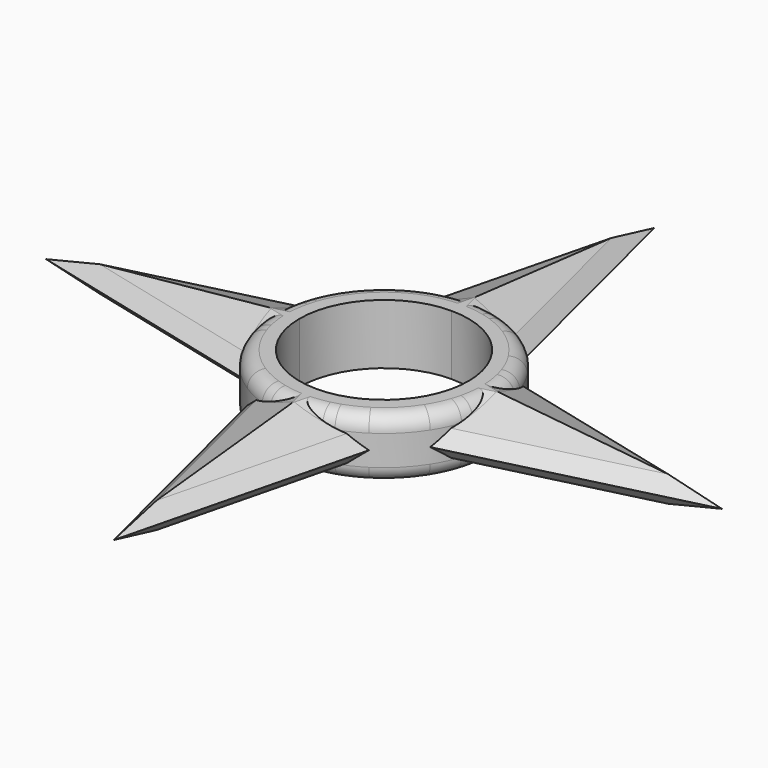
from build123d import *

# Parameters (mm, degrees)
F1_DEPTH      = 203.2
F2_SIZE       = 101.59999
F3_SIZE       = 81.28
F4_T2_ANGLE   = 24.7002002524
F4_T4_ANGLE   = 24.7002002524
F4_T6_ANGLE   = 24.7002002524
F4_T8_ANGLE   = 24.7002002524
F4_T10_ANGLE  = 24.7002002524
F4_T12_ANGLE  = 24.7002002524
F4_T14_ANGLE  = 24.7002002524
F4_T16_ANGLE  = 24.7002002524
F4_T20_ANGLE  = 19.2383475562
F4_T25_ANGLE  = 19.2383475562
F4_T30_ANGLE  = 19.2383475562
F4_T35_ANGLE  = 19.2383475562
F4_T40_ANGLE  = 19.2383475562
F4_T45_ANGLE  = 19.2383475562
F4_T50_ANGLE  = 19.2383475562
F4_T55_ANGLE  = 19.2383475562
F4_T60_ANGLE  = 19.2383475562
F4_T65_ANGLE  = 19.2383475562
F4_T70_ANGLE  = 19.2383475562
F4_T75_ANGLE  = 19.2383475562
F4_T80_ANGLE  = 19.2383475562
F4_T85_ANGLE  = 19.2383475562
F4_T90_ANGLE  = 19.2383475562
F4_T95_ANGLE  = 19.2383475562
F4_T100_ANGLE = 32.2106057484
F4_T105_ANGLE = 32.2106057484
F4_T110_ANGLE = 32.2106057484
F4_T115_ANGLE = 32.2106057484
F4_T120_ANGLE = 32.2106057484
F4_T125_ANGLE = 32.2106057484
F4_T130_ANGLE = 32.2106057484
F4_T135_ANGLE = 32.2106057484
F4_T140_ANGLE = 32.2106057484
F4_T145_ANGLE = 32.2106057484
F4_T150_ANGLE = 32.2106057484
F4_T155_ANGLE = 32.2106057484
F4_T160_ANGLE = 32.2106057484
F4_T165_ANGLE = 32.2106057484
F4_T170_ANGLE = 32.2106057484
F4_T175_ANGLE = 32.2106057484
F4_T180_ANGLE = 32.2106057484
F4_T185_ANGLE = 32.2106057484
F4_T190_ANGLE = 32.2106057484
F4_T195_ANGLE = 32.2106057484
F4_T200_ANGLE = 32.2106057484
F4_T205_ANGLE = 32.2106057484
F4_T210_ANGLE = 32.2106057484
F4_T215_ANGLE = 32.2106057484
F4_T220_ANGLE = 32.2106057484
F4_T225_ANGLE = 32.2106057484
F4_T230_ANGLE = 32.2106057484
F4_T235_ANGLE = 32.2106057484
F4_T240_ANGLE = 32.2106057484
F4_T245_ANGLE = 32.2106057484
F4_T250_ANGLE = 32.2106057484
F4_T255_ANGLE = 32.2106057484


# Not quite as in the source:
# - a fillet or chamfer that OpenCascade refuses, or shapes differently, is made with other operations: its cross-section is extruded or revolved along the edge and cut away or added
# - a fillet or chamfer is up to 0.001 mm smaller than in the source, because OpenCascade refuses the exact size


with BuildPart() as f1:
    # F0 (on Top) → F1 (new body)
    with BuildSketch(Plane.XY):
        with BuildLine():
            ThreePointArc((-205.551133263, 320.7954669478), (-107.0932469693, 365.6392162413), (0, 381))
            Line((0, 381), (0, 1143))
            Line((0, 1143), (-190.5, 381))
            Line((-190.5, 381), (-205.551133263, 320.7954669478))
        make_face()
        with BuildLine():
            Line((0, 1143), (0, 381))
            ThreePointArc((0, 381), (107.0932469693, 365.6392162413), (205.551133263, 320.7954669478))
            Line((205.551133263, 320.7954669478), (190.5, 381))
            Line((190.5, 381), (0, 1143))
        make_face()
        with BuildLine():
            Line((-1143, 0), (-381, 0))
            ThreePointArc((-381, 0), (-365.6392162413, 107.0932469693), (-320.7954669478, 205.551133263))
            Line((-320.7954669478, 205.551133263), (-381, 190.5))
            Line((-381, 190.5), (-1143, 0))
        make_face()
        with BuildLine():
            ThreePointArc((-320.7954669478, -205.551133263), (-365.6392162413, -107.0932469693), (-381, 0))
            Line((-381, 0), (-1143, 0))
            Line((-1143, 0), (-381, -190.5))
            Line((-381, -190.5), (-320.7954669478, -205.551133263))
        make_face()
        with BuildLine():
            Line((0, -1143), (0, -381))
            ThreePointArc((0, -381), (-107.0932469693, -365.6392162413), (-205.551133263, -320.7954669478))
            Line((-205.551133263, -320.7954669478), (-190.5, -381))
            Line((-190.5, -381), (0, -1143))
        make_face()
        with BuildLine():
            ThreePointArc((205.551133263, -320.7954669478), (107.0932469693, -365.6392162413), (0, -381))
            Line((0, -381), (0, -1143))
            Line((0, -1143), (190.5, -381))
            Line((190.5, -381), (205.551133263, -320.7954669478))
        make_face()
        with BuildLine():
            Line((1143, 0), (381, 0))
            ThreePointArc((381, 0), (365.6392162413, -107.0932469693), (320.7954669478, -205.551133263))
            Line((320.7954669478, -205.551133263), (381, -190.5))
            Line((381, -190.5), (1143, 0))
        make_face()
        with BuildLine():
            ThreePointArc((320.7954669478, 205.551133263), (365.6392162413, 107.0932469693), (381, 0))
            Line((381, 0), (1143, 0))
            Line((1143, 0), (381, 190.5))
            Line((381, 190.5), (320.7954669478, 205.551133263))
        make_face()
        with BuildLine():
            ThreePointArc((0, 292.1), (206.5458907846, 206.5458907846), (292.1, 0))
            Line((292.1, 0), (381, 0))
            ThreePointArc((381, 0), (365.6392162413, 107.0932469693), (320.7954669478, 205.551133263))
            ThreePointArc((320.7954669478, 205.551133263), (269.4076836321, 269.4076836321), (205.551133263, 320.7954669478))
            ThreePointArc((205.551133263, 320.7954669478), (107.0932469693, 365.6392162413), (0, 381))
            Line((0, 381), (0, 292.1))
        make_face()
        with BuildLine():
            ThreePointArc((-292.1, 0), (-206.5458907846, 206.5458907846), (0, 292.1))
            Line((0, 292.1), (0, 381))
            ThreePointArc((0, 381), (-107.0932469693, 365.6392162413), (-205.551133263, 320.7954669478))
            ThreePointArc((-205.551133263, 320.7954669478), (-269.4076836321, 269.4076836321), (-320.7954669478, 205.551133263))
            ThreePointArc((-320.7954669478, 205.551133263), (-365.6392162413, 107.0932469693), (-381, 0))
            Line((-381, 0), (-292.1, 0))
        make_face()
        with BuildLine():
            Line((381, 0), (292.1, 0))
            ThreePointArc((292.1, 0), (206.5458907846, -206.5458907846), (0, -292.1))
            Line((0, -292.1), (0, -381))
            ThreePointArc((0, -381), (107.0932469693, -365.6392162413), (205.551133263, -320.7954669478))
            ThreePointArc((205.551133263, -320.7954669478), (269.4076836321, -269.4076836321), (320.7954669478, -205.551133263))
            ThreePointArc((320.7954669478, -205.551133263), (365.6392162413, -107.0932469693), (381, 0))
        make_face()
        with BuildLine():
            ThreePointArc((-292.1, 0), (-206.5458907846, -206.5458907846), (0, -292.1))
            Line((0, -292.1), (0, -285.75))
            ThreePointArc((0, -285.75), (-202.0557627241, -202.0557627241), (-285.75, 0))
            Line((-285.75, 0), (-292.1, 0))
        make_face()
        with BuildLine():
            Line((0, 285.75), (0, 292.1))
            ThreePointArc((0, 292.1), (-206.5458907846, 206.5458907846), (-292.1, 0))
            Line((-292.1, 0), (-285.75, 0))
            ThreePointArc((-285.75, 0), (-202.0557627241, 202.0557627241), (0, 285.75))
        make_face()
        with BuildLine():
            ThreePointArc((0, -292.1), (206.5458907846, -206.5458907846), (292.1, 0))
            Line((292.1, 0), (285.75, 0))
            ThreePointArc((285.75, 0), (202.0557627241, -202.0557627241), (0, -285.75))
            Line((0, -285.75), (0, -292.1))
        make_face()
        with BuildLine():
            Line((285.75, 0), (292.1, 0))
            ThreePointArc((292.1, 0), (206.5458907846, 206.5458907846), (0, 292.1))
            Line((0, 292.1), (0, 285.75))
            ThreePointArc((0, 285.75), (202.0557627241, 202.0557627241), (285.75, 0))
        make_face()
        with BuildLine():
            Line((0, -381), (0, -292.1))
            ThreePointArc((0, -292.1), (-206.5458907846, -206.5458907846), (-292.1, 0))
            Line((-292.1, 0), (-381, 0))
            ThreePointArc((-381, 0), (-365.6392162413, -107.0932469693), (-320.7954669478, -205.551133263))
            ThreePointArc((-320.7954669478, -205.551133263), (-269.4076836321, -269.4076836321), (-205.551133263, -320.7954669478))
            ThreePointArc((-205.551133263, -320.7954669478), (-107.0932469693, -365.6392162413), (0, -381))
        make_face()
    extrude(amount=F1_DEPTH)

    # F2 (size 101.6 in the source; OpenCascade refuses exactly that, so slightly less here)
    f2_edges = [f1.edges().sort_by_distance(p)[0] for p in [
        (-731.897733, -102.775567, 203.2),
        (-731.897733, -102.775567, 0),
        (-731.897733, 102.775567, 203.2),
        (-731.897733, 102.775567, 0),
        (-102.775567, 731.897733, 203.2),
        (-102.775567, 731.897733, 0),
        (102.775567, 731.897733, 203.2),
        (102.775567, 731.897733, 0),
        (731.897733, 102.775567, 203.2),
        (731.897733, 102.775567, 0),
        (731.897733, -102.775567, 203.2),
        (731.897733, -102.775567, 0),
        (102.775567, -731.897733, 203.2),
        (102.775567, -731.897733, 0),
        (-102.775567, -731.897733, 203.2),
        (-102.775567, -731.897733, 0),
    ]]
    chamfer(f2_edges, length=F2_SIZE)

    # F3
    f3_edges = [f1.edges().sort_by_distance(p)[0] for p in [
        (-44.185339, -547.351154, 203.2),
        (44.185339, -547.351154, 203.2),
        (547.351154, -44.185339, 203.2),
        (547.351154, 44.185339, 203.2),
        (44.185339, 547.351154, 203.2),
        (-44.185339, 547.351154, 203.2),
        (-547.351154, 44.185339, 203.2),
        (-547.351154, -44.185339, 203.2),
        (-44.185339, 547.351154, 0),
        (44.185339, 547.351154, 0),
        (547.351154, 44.185339, 0),
        (547.351154, -44.185339, 0),
        (44.185339, -547.351154, 0),
        (-44.185339, -547.351154, 0),
        (-547.351154, 44.185339, 0),
        (-547.351154, -44.185339, 0),
    ]]
    chamfer(f3_edges, length=F3_SIZE)

    # F4: fillet of radius 50.8 on 24 edges, made by hand

    # F4_s1 → F4_t2 (revolve, cut)
    with BuildSketch(Plane(origin=(0, 0, 0), x_dir=(0, 0, 1), z_dir=(0.8419828529, 0.5395042868, 0))):
        with BuildLine():
            ThreePointArc((0, -330.2), (14.8789755157, -366.1210244843), (50.8, -381))
            Line((50.8, -381), (0, -381))
            Line((0, -381), (0, -330.2))
        make_face()
    revolve(axis=Axis((0, 0, 0), (0, 0, 1)), revolution_arc=F4_T2_ANGLE, mode=Mode.SUBTRACT)

    # F4_s3 → F4_t4 (revolve, cut)
    with BuildSketch(Plane(origin=(0, 0, 0), x_dir=(0, 0, 1), z_dir=(0.8419828529, 0.5395042868, 0))):
        with BuildLine():
            ThreePointArc((203.2, -330.2), (188.3210244843, -366.1210244843), (152.4, -381))
            Line((152.4, -381), (203.2, -381))
            Line((203.2, -381), (203.2, -330.2))
        make_face()
    revolve(axis=Axis((0, 0, 203.2), (0, 0, 1)), revolution_arc=F4_T4_ANGLE, mode=Mode.SUBTRACT)

    # F4_s5 → F4_t6 (revolve, cut)
    with BuildSketch(Plane(origin=(0, 0, 0), x_dir=(0, 0, 1), z_dir=(0.5395042868, -0.8419828529, 0))):
        with BuildLine():
            ThreePointArc((0, -330.2), (14.8789755157, -366.1210244843), (50.8, -381))
            Line((50.8, -381), (0, -381))
            Line((0, -381), (0, -330.2))
        make_face()
    revolve(axis=Axis((0, 0, 0), (0, 0, 1)), revolution_arc=F4_T6_ANGLE, mode=Mode.SUBTRACT)

    # F4_s7 → F4_t8 (revolve, cut)
    with BuildSketch(Plane(origin=(0, 0, 0), x_dir=(0, 0, 1), z_dir=(0.5395042868, -0.8419828529, 0))):
        with BuildLine():
            ThreePointArc((203.2, -330.2), (188.3210244843, -366.1210244843), (152.4, -381))
            Line((152.4, -381), (203.2, -381))
            Line((203.2, -381), (203.2, -330.2))
        make_face()
    revolve(axis=Axis((0, 0, 203.2), (0, 0, 1)), revolution_arc=F4_T8_ANGLE, mode=Mode.SUBTRACT)

    # F4_s9 → F4_t10 (revolve, cut)
    with BuildSketch(Plane(origin=(0, 0, 0), x_dir=(0, 0, 1), z_dir=(-0.8419828529, -0.5395042868, 0))):
        with BuildLine():
            ThreePointArc((0, -330.2), (14.8789755157, -366.1210244843), (50.8, -381))
            Line((50.8, -381), (0, -381))
            Line((0, -381), (0, -330.2))
        make_face()
    revolve(axis=Axis((0, 0, 0), (0, 0, 1)), revolution_arc=F4_T10_ANGLE, mode=Mode.SUBTRACT)

    # F4_s11 → F4_t12 (revolve, cut)
    with BuildSketch(Plane(origin=(0, 0, 0), x_dir=(0, 0, 1), z_dir=(-0.8419828529, -0.5395042868, 0))):
        with BuildLine():
            ThreePointArc((203.2, -330.2), (188.3210244843, -366.1210244843), (152.4, -381))
            Line((152.4, -381), (203.2, -381))
            Line((203.2, -381), (203.2, -330.2))
        make_face()
    revolve(axis=Axis((0, 0, 203.2), (0, 0, 1)), revolution_arc=F4_T12_ANGLE, mode=Mode.SUBTRACT)

    # F4_s13 → F4_t14 (revolve, cut)
    with BuildSketch(Plane(origin=(0, 0, 0), x_dir=(0, 0, 1), z_dir=(-0.5395042868, 0.8419828529, 0))):
        with BuildLine():
            ThreePointArc((50.8, -381), (14.8789755157, -366.1210244843), (0, -330.2))
            Line((0, -330.2), (0, -381))
            Line((0, -381), (50.8, -381))
        make_face()
    revolve(axis=Axis((0, 0, 0), (0, 0, 1)), revolution_arc=F4_T14_ANGLE, mode=Mode.SUBTRACT)

    # F4_s15 → F4_t16 (revolve, cut)
    with BuildSketch(Plane(origin=(0, 0, 0), x_dir=(0, 0, 1), z_dir=(-0.5395042868, 0.8419828529, 0))):
        with BuildLine():
            ThreePointArc((152.4, -381), (188.3210244843, -366.1210244843), (203.2, -330.2))
            Line((203.2, -330.2), (203.2, -381))
            Line((203.2, -381), (152.4, -381))
        make_face()
    revolve(axis=Axis((0, 0, 203.2), (0, 0, 1)), revolution_arc=F4_T16_ANGLE, mode=Mode.SUBTRACT)


with BuildPart() as f4_tool18:
    # F4_s19 → F4_t20 (revolve)
    with BuildSketch(Plane(origin=(0, 0, 0), x_dir=(0, 0, 1), z_dir=(0.5395042868, -0.8419828529, 0))):
        with BuildLine():
            ThreePointArc((50.8, 381), (14.8789755157, 366.1210244843), (0, 330.2))
            Line((0, 330.2), (0, 381))
            Line((0, 381), (50.8, 381))
        make_face()
    revolve(axis=Axis((0, 0, 0), (0, 0, -1)), revolution_arc=F4_T20_ANGLE)

    split(bisect_by=Plane(origin=(-3.3507542833, -13.4030171331, -33.3536008728), x_dir=(0.9701425001, -0.242535625, 0), z_dir=(-0.0928143655, -0.3712574618, -0.9238795325)), keep=Keep.TOP)


with BuildPart() as f1_1:
    add(f1.part)

    # F4_t17: cut F4_tool18
    add(f4_tool18.part, mode=Mode.SUBTRACT)


with BuildPart() as f4_tool23:
    # F4_s24 → F4_t25 (revolve)
    with BuildSketch(Plane(origin=(0, 0, 0), x_dir=(0, 0, 1), z_dir=(-0.8419828529, 0.5395042868, 0))):
        with BuildLine():
            ThreePointArc((50.8, -381), (14.8789755157, -366.1210244843), (0, -330.2))
            Line((0, -330.2), (0, -381))
            Line((0, -381), (50.8, -381))
        make_face()
    revolve(axis=Axis((0, 0, 0), (0, 0, 1)), revolution_arc=F4_T25_ANGLE)

    split(bisect_by=Plane(origin=(-13.4030171331, -3.3507542833, -33.3536008728), x_dir=(0.242535625, -0.9701425001, 0), z_dir=(-0.3712574618, -0.0928143655, -0.9238795325)), keep=Keep.TOP)


with BuildPart() as f1_2:
    add(f1_1.part)

    # F4_t22: cut F4_tool23
    add(f4_tool23.part, mode=Mode.SUBTRACT)


with BuildPart() as f4_tool28:
    # F4_s29 → F4_t30 (revolve)
    with BuildSketch(Plane(origin=(0, 0, 0), x_dir=(0, 0, 1), z_dir=(0.5395042868, -0.8419828529, 0))):
        with BuildLine():
            ThreePointArc((152.4, 381), (188.3210244843, 366.1210244843), (203.2, 330.2))
            Line((203.2, 330.2), (203.2, 381))
            Line((203.2, 381), (152.4, 381))
        make_face()
    revolve(axis=Axis((0, 0, 203.2), (0, 0, -1)), revolution_arc=F4_T30_ANGLE)

    split(bisect_by=Plane(origin=(-20.7750105338, -83.1000421351, 206.7956498413), x_dir=(0.9701425001, -0.242535625, 0), z_dir=(-0.0928143655, -0.3712574618, 0.9238795325)), keep=Keep.TOP)


with BuildPart() as f1_3:
    add(f1_2.part)

    # F4_t27: cut F4_tool28
    add(f4_tool28.part, mode=Mode.SUBTRACT)


with BuildPart() as f4_tool33:
    # F4_s34 → F4_t35 (revolve)
    with BuildSketch(Plane(origin=(0, 0, 0), x_dir=(0, 0, 1), z_dir=(-0.8419828529, 0.5395042868, 0))):
        with BuildLine():
            ThreePointArc((152.4, -381), (188.3210244843, -366.1210244843), (203.2, -330.2))
            Line((203.2, -330.2), (203.2, -381))
            Line((203.2, -381), (152.4, -381))
        make_face()
    revolve(axis=Axis((0, 0, 203.2), (0, 0, 1)), revolution_arc=F4_T35_ANGLE)

    split(bisect_by=Plane(origin=(-83.1000421351, -20.7750105338, 206.7956498413), x_dir=(0.242535625, -0.9701425001, 0), z_dir=(-0.3712574618, -0.0928143655, 0.9238795325)), keep=Keep.TOP)


with BuildPart() as f1_4:
    add(f1_3.part)

    # F4_t32: cut F4_tool33
    add(f4_tool33.part, mode=Mode.SUBTRACT)


with BuildPart() as f4_tool38:
    # F4_s39 → F4_t40 (revolve)
    with BuildSketch(Plane(origin=(0, 0, 0), x_dir=(0, 0, 1), z_dir=(-0.8419828529, -0.5395042868, 0))):
        with BuildLine():
            ThreePointArc((0, 330.2), (14.8789755157, 366.1210244843), (50.8, 381))
            Line((50.8, 381), (0, 381))
            Line((0, 381), (0, 330.2))
        make_face()
    revolve(axis=Axis((0, 0, 0), (0, 0, -1)), revolution_arc=F4_T40_ANGLE)

    split(bisect_by=Plane(origin=(-13.4030171331, 3.3507542833, -33.3536008728), x_dir=(-0.242535625, -0.9701425001, 0), z_dir=(-0.3712574618, 0.0928143655, -0.9238795325)), keep=Keep.TOP)


with BuildPart() as f1_5:
    add(f1_4.part)

    # F4_t37: cut F4_tool38
    add(f4_tool38.part, mode=Mode.SUBTRACT)


with BuildPart() as f4_tool43:
    # F4_s44 → F4_t45 (revolve)
    with BuildSketch(Plane(origin=(0, 0, 0), x_dir=(0, 0, 1), z_dir=(0.5395042868, 0.8419828529, 0))):
        with BuildLine():
            ThreePointArc((0, -330.2), (14.8789755157, -366.1210244843), (50.8, -381))
            Line((50.8, -381), (0, -381))
            Line((0, -381), (0, -330.2))
        make_face()
    revolve(axis=Axis((0, 0, 0), (0, 0, 1)), revolution_arc=F4_T45_ANGLE)

    split(bisect_by=Plane(origin=(-3.3507542833, 13.4030171331, -33.3536008728), x_dir=(-0.9701425001, -0.242535625, 0), z_dir=(-0.0928143655, 0.3712574618, -0.9238795325)), keep=Keep.TOP)


with BuildPart() as f1_6:
    add(f1_5.part)

    # F4_t42: cut F4_tool43
    add(f4_tool43.part, mode=Mode.SUBTRACT)


with BuildPart() as f4_tool48:
    # F4_s49 → F4_t50 (revolve)
    with BuildSketch(Plane(origin=(0, 0, 0), x_dir=(0, 0, 1), z_dir=(0.8419828529, -0.5395042868, 0))):
        with BuildLine():
            ThreePointArc((0, -330.2), (14.8789755157, -366.1210244843), (50.8, -381))
            Line((50.8, -381), (0, -381))
            Line((0, -381), (0, -330.2))
        make_face()
    revolve(axis=Axis((0, 0, 0), (0, 0, 1)), revolution_arc=F4_T50_ANGLE)

    split(bisect_by=Plane(origin=(13.4030171331, 3.3507542833, -33.3536008728), x_dir=(-0.242535625, 0.9701425001, 0), z_dir=(0.3712574618, 0.0928143655, -0.9238795325)), keep=Keep.TOP)


with BuildPart() as f1_7:
    add(f1_6.part)

    # F4_t47: cut F4_tool48
    add(f4_tool48.part, mode=Mode.SUBTRACT)


with BuildPart() as f4_tool53:
    # F4_s54 → F4_t55 (revolve)
    with BuildSketch(Plane(origin=(0, 0, 0), x_dir=(0, 0, 1), z_dir=(-0.5395042868, 0.8419828529, 0))):
        with BuildLine():
            ThreePointArc((0, 330.2), (14.8789755157, 366.1210244843), (50.8, 381))
            Line((50.8, 381), (0, 381))
            Line((0, 381), (0, 330.2))
        make_face()
    revolve(axis=Axis((0, 0, 0), (0, 0, -1)), revolution_arc=F4_T55_ANGLE)

    split(bisect_by=Plane(origin=(3.3507542833, 13.4030171331, -33.3536008728), x_dir=(-0.9701425001, 0.242535625, 0), z_dir=(0.0928143655, 0.3712574618, -0.9238795325)), keep=Keep.TOP)


with BuildPart() as f1_8:
    add(f1_7.part)

    # F4_t52: cut F4_tool53
    add(f4_tool53.part, mode=Mode.SUBTRACT)


with BuildPart() as f4_tool58:
    # F4_s59 → F4_t60 (revolve)
    with BuildSketch(Plane(origin=(0, 0, 0), x_dir=(0, 0, 1), z_dir=(-0.5395042868, -0.8419828529, 0))):
        with BuildLine():
            ThreePointArc((0, -330.2), (14.8789755157, -366.1210244843), (50.8, -381))
            Line((50.8, -381), (0, -381))
            Line((0, -381), (0, -330.2))
        make_face()
    revolve(axis=Axis((0, 0, 0), (0, 0, 1)), revolution_arc=F4_T60_ANGLE)

    split(bisect_by=Plane(origin=(3.3507542833, -13.4030171331, -33.3536008728), x_dir=(0.9701425001, 0.242535625, 0), z_dir=(0.0928143655, -0.3712574618, -0.9238795325)), keep=Keep.TOP)


with BuildPart() as f1_9:
    add(f1_8.part)

    # F4_t57: cut F4_tool58
    add(f4_tool58.part, mode=Mode.SUBTRACT)


with BuildPart() as f4_tool63:
    # F4_s64 → F4_t65 (revolve)
    with BuildSketch(Plane(origin=(0, 0, 0), x_dir=(0, 0, 1), z_dir=(0.8419828529, 0.5395042868, 0))):
        with BuildLine():
            ThreePointArc((0, 330.2), (14.8789755157, 366.1210244843), (50.8, 381))
            Line((50.8, 381), (0, 381))
            Line((0, 381), (0, 330.2))
        make_face()
    revolve(axis=Axis((0, 0, 0), (0, 0, -1)), revolution_arc=F4_T65_ANGLE)

    split(bisect_by=Plane(origin=(13.4030171331, -3.3507542833, -33.3536008728), x_dir=(0.242535625, 0.9701425001, 0), z_dir=(0.3712574618, -0.0928143655, -0.9238795325)), keep=Keep.TOP)


with BuildPart() as f1_10:
    add(f1_9.part)

    # F4_t62: cut F4_tool63
    add(f4_tool63.part, mode=Mode.SUBTRACT)


with BuildPart() as f4_tool68:
    # F4_s69 → F4_t70 (revolve)
    with BuildSketch(Plane(origin=(0, 0, 0), x_dir=(0, 0, 1), z_dir=(0.8419828529, 0.5395042868, 0))):
        with BuildLine():
            ThreePointArc((203.2, 330.2), (188.3210244843, 366.1210244843), (152.4, 381))
            Line((152.4, 381), (203.2, 381))
            Line((203.2, 381), (203.2, 330.2))
        make_face()
    revolve(axis=Axis((0, 0, 203.2), (0, 0, -1)), revolution_arc=F4_T70_ANGLE)

    split(bisect_by=Plane(origin=(83.1000421351, -20.7750105338, 206.7956498413), x_dir=(0.242535625, 0.9701425001, 0), z_dir=(0.3712574618, -0.0928143655, 0.9238795325)), keep=Keep.TOP)


with BuildPart() as f1_11:
    add(f1_10.part)

    # F4_t67: cut F4_tool68
    add(f4_tool68.part, mode=Mode.SUBTRACT)


with BuildPart() as f4_tool73:
    # F4_s74 → F4_t75 (revolve)
    with BuildSketch(Plane(origin=(0, 0, 0), x_dir=(0, 0, 1), z_dir=(-0.5395042868, -0.8419828529, 0))):
        with BuildLine():
            ThreePointArc((203.2, -330.2), (188.3210244843, -366.1210244843), (152.4, -381))
            Line((152.4, -381), (203.2, -381))
            Line((203.2, -381), (203.2, -330.2))
        make_face()
    revolve(axis=Axis((0, 0, 203.2), (0, 0, 1)), revolution_arc=F4_T75_ANGLE)

    split(bisect_by=Plane(origin=(20.7750105338, -83.1000421351, 206.7956498413), x_dir=(0.9701425001, 0.242535625, 0), z_dir=(0.0928143655, -0.3712574618, 0.9238795325)), keep=Keep.TOP)


with BuildPart() as f1_12:
    add(f1_11.part)

    # F4_t72: cut F4_tool73
    add(f4_tool73.part, mode=Mode.SUBTRACT)


with BuildPart() as f4_tool78:
    # F4_s79 → F4_t80 (revolve)
    with BuildSketch(Plane(origin=(0, 0, 0), x_dir=(0, 0, 1), z_dir=(0.5395042868, 0.8419828529, 0))):
        with BuildLine():
            ThreePointArc((203.2, -330.2), (188.3210244843, -366.1210244843), (152.4, -381))
            Line((152.4, -381), (203.2, -381))
            Line((203.2, -381), (203.2, -330.2))
        make_face()
    revolve(axis=Axis((0, 0, 203.2), (0, 0, 1)), revolution_arc=F4_T80_ANGLE)

    split(bisect_by=Plane(origin=(-20.7750105338, 83.1000421351, 206.7956498413), x_dir=(-0.9701425001, -0.242535625, 0), z_dir=(-0.0928143655, 0.3712574618, 0.9238795325)), keep=Keep.TOP)


with BuildPart() as f1_13:
    add(f1_12.part)

    # F4_t77: cut F4_tool78
    add(f4_tool78.part, mode=Mode.SUBTRACT)


with BuildPart() as f4_tool83:
    # F4_s84 → F4_t85 (revolve)
    with BuildSketch(Plane(origin=(0, 0, 0), x_dir=(0, 0, 1), z_dir=(-0.8419828529, -0.5395042868, 0))):
        with BuildLine():
            ThreePointArc((203.2, 330.2), (188.3210244843, 366.1210244843), (152.4, 381))
            Line((152.4, 381), (203.2, 381))
            Line((203.2, 381), (203.2, 330.2))
        make_face()
    revolve(axis=Axis((0, 0, 203.2), (0, 0, -1)), revolution_arc=F4_T85_ANGLE)

    split(bisect_by=Plane(origin=(-83.1000421351, 20.7750105338, 206.7956498413), x_dir=(-0.242535625, -0.9701425001, 0), z_dir=(-0.3712574618, 0.0928143655, 0.9238795325)), keep=Keep.TOP)


with BuildPart() as f1_14:
    add(f1_13.part)

    # F4_t82: cut F4_tool83
    add(f4_tool83.part, mode=Mode.SUBTRACT)


with BuildPart() as f4_tool88:
    # F4_s89 → F4_t90 (revolve)
    with BuildSketch(Plane(origin=(0, 0, 0), x_dir=(0, 0, 1), z_dir=(-0.5395042868, 0.8419828529, 0))):
        with BuildLine():
            ThreePointArc((203.2, 330.2), (188.3210244843, 366.1210244843), (152.4, 381))
            Line((152.4, 381), (203.2, 381))
            Line((203.2, 381), (203.2, 330.2))
        make_face()
    revolve(axis=Axis((0, 0, 203.2), (0, 0, -1)), revolution_arc=F4_T90_ANGLE)

    split(bisect_by=Plane(origin=(20.7750105338, 83.1000421351, 206.7956498413), x_dir=(-0.9701425001, 0.242535625, 0), z_dir=(0.0928143655, 0.3712574618, 0.9238795325)), keep=Keep.TOP)


with BuildPart() as f1_15:
    add(f1_14.part)

    # F4_t87: cut F4_tool88
    add(f4_tool88.part, mode=Mode.SUBTRACT)


with BuildPart() as f4_tool93:
    # F4_s94 → F4_t95 (revolve)
    with BuildSketch(Plane(origin=(0, 0, 0), x_dir=(0, 0, 1), z_dir=(0.8419828529, -0.5395042868, 0))):
        with BuildLine():
            ThreePointArc((203.2, -330.2), (188.3210244843, -366.1210244843), (152.4, -381))
            Line((152.4, -381), (203.2, -381))
            Line((203.2, -381), (203.2, -330.2))
        make_face()
    revolve(axis=Axis((0, 0, 203.2), (0, 0, 1)), revolution_arc=F4_T95_ANGLE)

    split(bisect_by=Plane(origin=(83.1000421351, 20.7750105338, 206.7956498413), x_dir=(-0.242535625, 0.9701425001, 0), z_dir=(0.3712574618, 0.0928143655, 0.9238795325)), keep=Keep.TOP)


with BuildPart() as f1_16:
    add(f1_15.part)

    # F4_t92: cut F4_tool93
    add(f4_tool93.part, mode=Mode.SUBTRACT)


with BuildPart() as f4_tool98:
    # F4_s99 → F4_t100 (revolve)
    with BuildSketch(Plane(origin=(0, 0, 0), x_dir=(0, 0, 1), z_dir=(0.972729132, -0.2319440357, 0))):
        with BuildLine():
            ThreePointArc((203.2, -330.2), (188.3210244843, -366.1210244843), (152.4, -381))
            Line((152.4, -381), (203.2, -381))
            Line((203.2, -381), (203.2, -330.2))
        make_face()
    revolve(axis=Axis((0, 0, 203.2), (0, 0, 1)), revolution_arc=F4_T100_ANGLE)

    split(bisect_by=Plane(origin=(83.1000421351, 20.7750105338, 206.7956498413), x_dir=(-0.242535625, 0.9701425001, 0), z_dir=(0.3712574618, 0.0928143655, 0.9238795325)), keep=Keep.TOP)


with BuildPart() as f1_17:
    add(f1_16.part)

    # F4_t97: cut F4_tool98
    add(f4_tool98.part, mode=Mode.SUBTRACT)


with BuildPart() as f4_tool103:
    # F4_s104 → F4_t105 (revolve)
    with BuildSketch(Plane(origin=(0, 0, 0), x_dir=(0, 0, 1), z_dir=(0.972729132, -0.2319440357, 0))):
        with BuildLine():
            ThreePointArc((203.2, -330.2), (188.3210244843, -366.1210244843), (152.4, -381))
            Line((152.4, -381), (203.2, -381))
            Line((203.2, -381), (203.2, -330.2))
        make_face()
    revolve(axis=Axis((0, 0, 203.2), (0, 0, 1)), revolution_arc=F4_T105_ANGLE)

    split(bisect_by=Plane(origin=(-83.1000421351, 20.7750105338, 206.7956498413), x_dir=(-0.242535625, -0.9701425001, 0), z_dir=(-0.3712574618, 0.0928143655, 0.9238795325)), keep=Keep.TOP)


with BuildPart() as f1_18:
    add(f1_17.part)

    # F4_t102: cut F4_tool103
    add(f4_tool103.part, mode=Mode.SUBTRACT)


with BuildPart() as f4_tool108:
    # F4_s109 → F4_t110 (revolve)
    with BuildSketch(Plane(origin=(0, 0, 0), x_dir=(0, 0, 1), z_dir=(-0.2319440357, 0.972729132, 0))):
        with BuildLine():
            ThreePointArc((203.2, 330.2), (188.3210244843, 366.1210244843), (152.4, 381))
            Line((152.4, 381), (203.2, 381))
            Line((203.2, 381), (203.2, 330.2))
        make_face()
    revolve(axis=Axis((0, 0, 203.2), (0, 0, -1)), revolution_arc=F4_T110_ANGLE)

    split(bisect_by=Plane(origin=(20.7750105338, 83.1000421351, 206.7956498413), x_dir=(-0.9701425001, 0.242535625, 0), z_dir=(0.0928143655, 0.3712574618, 0.9238795325)), keep=Keep.TOP)


with BuildPart() as f1_19:
    add(f1_18.part)

    # F4_t107: cut F4_tool108
    add(f4_tool108.part, mode=Mode.SUBTRACT)


with BuildPart() as f4_tool113:
    # F4_s114 → F4_t115 (revolve)
    with BuildSketch(Plane(origin=(0, 0, 0), x_dir=(0, 0, 1), z_dir=(-0.2319440357, 0.972729132, 0))):
        with BuildLine():
            ThreePointArc((203.2, 330.2), (188.3210244843, 366.1210244843), (152.4, 381))
            Line((152.4, 381), (203.2, 381))
            Line((203.2, 381), (203.2, 330.2))
        make_face()
    revolve(axis=Axis((0, 0, 203.2), (0, 0, -1)), revolution_arc=F4_T115_ANGLE)

    split(bisect_by=Plane(origin=(20.7750105338, -83.1000421351, 206.7956498413), x_dir=(0.9701425001, 0.242535625, 0), z_dir=(0.0928143655, -0.3712574618, 0.9238795325)), keep=Keep.TOP)


with BuildPart() as f1_20:
    add(f1_19.part)

    # F4_t112: cut F4_tool113
    add(f4_tool113.part, mode=Mode.SUBTRACT)


with BuildPart() as f4_tool118:
    # F4_s119 → F4_t120 (revolve)
    with BuildSketch(Plane(origin=(0, 0, 0), x_dir=(0, 0, 1), z_dir=(-0.972729132, -0.2319440357, 0))):
        with BuildLine():
            ThreePointArc((203.2, 330.2), (188.3210244843, 366.1210244843), (152.4, 381))
            Line((152.4, 381), (203.2, 381))
            Line((203.2, 381), (203.2, 330.2))
        make_face()
    revolve(axis=Axis((0, 0, 203.2), (0, 0, -1)), revolution_arc=F4_T120_ANGLE)

    split(bisect_by=Plane(origin=(-83.1000421351, 20.7750105338, 206.7956498413), x_dir=(-0.242535625, -0.9701425001, 0), z_dir=(-0.3712574618, 0.0928143655, 0.9238795325)), keep=Keep.TOP)


with BuildPart() as f1_21:
    add(f1_20.part)

    # F4_t117: cut F4_tool118
    add(f4_tool118.part, mode=Mode.SUBTRACT)


with BuildPart() as f4_tool123:
    # F4_s124 → F4_t125 (revolve)
    with BuildSketch(Plane(origin=(0, 0, 0), x_dir=(0, 0, 1), z_dir=(-0.972729132, -0.2319440357, 0))):
        with BuildLine():
            ThreePointArc((203.2, 330.2), (188.3210244843, 366.1210244843), (152.4, 381))
            Line((152.4, 381), (203.2, 381))
            Line((203.2, 381), (203.2, 330.2))
        make_face()
    revolve(axis=Axis((0, 0, 203.2), (0, 0, -1)), revolution_arc=F4_T125_ANGLE)

    split(bisect_by=Plane(origin=(83.1000421351, 20.7750105338, 206.7956498413), x_dir=(-0.242535625, 0.9701425001, 0), z_dir=(0.3712574618, 0.0928143655, 0.9238795325)), keep=Keep.TOP)


with BuildPart() as f1_22:
    add(f1_21.part)

    # F4_t122: cut F4_tool123
    add(f4_tool123.part, mode=Mode.SUBTRACT)


with BuildPart() as f4_tool128:
    # F4_s129 → F4_t130 (revolve)
    with BuildSketch(Plane(origin=(0, 0, 0), x_dir=(0, 0, 1), z_dir=(0.2319440357, 0.972729132, 0))):
        with BuildLine():
            ThreePointArc((203.2, -330.2), (188.3210244843, -366.1210244843), (152.4, -381))
            Line((152.4, -381), (203.2, -381))
            Line((203.2, -381), (203.2, -330.2))
        make_face()
    revolve(axis=Axis((0, 0, 203.2), (0, 0, 1)), revolution_arc=F4_T130_ANGLE)

    split(bisect_by=Plane(origin=(-20.7750105338, 83.1000421351, 206.7956498413), x_dir=(-0.9701425001, -0.242535625, 0), z_dir=(-0.0928143655, 0.3712574618, 0.9238795325)), keep=Keep.TOP)


with BuildPart() as f1_23:
    add(f1_22.part)

    # F4_t127: cut F4_tool128
    add(f4_tool128.part, mode=Mode.SUBTRACT)


with BuildPart() as f4_tool133:
    # F4_s134 → F4_t135 (revolve)
    with BuildSketch(Plane(origin=(0, 0, 0), x_dir=(0, 0, 1), z_dir=(0.2319440357, 0.972729132, 0))):
        with BuildLine():
            ThreePointArc((203.2, -330.2), (188.3210244843, -366.1210244843), (152.4, -381))
            Line((152.4, -381), (203.2, -381))
            Line((203.2, -381), (203.2, -330.2))
        make_face()
    revolve(axis=Axis((0, 0, 203.2), (0, 0, 1)), revolution_arc=F4_T135_ANGLE)

    split(bisect_by=Plane(origin=(-20.7750105338, -83.1000421351, 206.7956498413), x_dir=(0.9701425001, -0.242535625, 0), z_dir=(-0.0928143655, -0.3712574618, 0.9238795325)), keep=Keep.TOP)


with BuildPart() as f1_24:
    add(f1_23.part)

    # F4_t132: cut F4_tool133
    add(f4_tool133.part, mode=Mode.SUBTRACT)


with BuildPart() as f4_tool138:
    # F4_s139 → F4_t140 (revolve)
    with BuildSketch(Plane(origin=(0, 0, 0), x_dir=(0, 0, 1), z_dir=(-0.2319440357, -0.972729132, 0))):
        with BuildLine():
            ThreePointArc((203.2, -330.2), (188.3210244843, -366.1210244843), (152.4, -381))
            Line((152.4, -381), (203.2, -381))
            Line((203.2, -381), (203.2, -330.2))
        make_face()
    revolve(axis=Axis((0, 0, 203.2), (0, 0, 1)), revolution_arc=F4_T140_ANGLE)

    split(bisect_by=Plane(origin=(20.7750105338, -83.1000421351, 206.7956498413), x_dir=(0.9701425001, 0.242535625, 0), z_dir=(0.0928143655, -0.3712574618, 0.9238795325)), keep=Keep.TOP)


with BuildPart() as f1_25:
    add(f1_24.part)

    # F4_t137: cut F4_tool138
    add(f4_tool138.part, mode=Mode.SUBTRACT)


with BuildPart() as f4_tool143:
    # F4_s144 → F4_t145 (revolve)
    with BuildSketch(Plane(origin=(0, 0, 0), x_dir=(0, 0, 1), z_dir=(-0.2319440357, -0.972729132, 0))):
        with BuildLine():
            ThreePointArc((203.2, -330.2), (188.3210244843, -366.1210244843), (152.4, -381))
            Line((152.4, -381), (203.2, -381))
            Line((203.2, -381), (203.2, -330.2))
        make_face()
    revolve(axis=Axis((0, 0, 203.2), (0, 0, 1)), revolution_arc=F4_T145_ANGLE)

    split(bisect_by=Plane(origin=(20.7750105338, 83.1000421351, 206.7956498413), x_dir=(-0.9701425001, 0.242535625, 0), z_dir=(0.0928143655, 0.3712574618, 0.9238795325)), keep=Keep.TOP)


with BuildPart() as f1_26:
    add(f1_25.part)

    # F4_t142: cut F4_tool143
    add(f4_tool143.part, mode=Mode.SUBTRACT)


with BuildPart() as f4_tool148:
    # F4_s149 → F4_t150 (revolve)
    with BuildSketch(Plane(origin=(0, 0, 0), x_dir=(0, 0, 1), z_dir=(0.972729132, 0.2319440357, 0))):
        with BuildLine():
            ThreePointArc((203.2, 330.2), (188.3210244843, 366.1210244843), (152.4, 381))
            Line((152.4, 381), (203.2, 381))
            Line((203.2, 381), (203.2, 330.2))
        make_face()
    revolve(axis=Axis((0, 0, 203.2), (0, 0, -1)), revolution_arc=F4_T150_ANGLE)

    split(bisect_by=Plane(origin=(83.1000421351, -20.7750105338, 206.7956498413), x_dir=(0.242535625, 0.9701425001, 0), z_dir=(0.3712574618, -0.0928143655, 0.9238795325)), keep=Keep.TOP)


with BuildPart() as f1_27:
    add(f1_26.part)

    # F4_t147: cut F4_tool148
    add(f4_tool148.part, mode=Mode.SUBTRACT)


with BuildPart() as f4_tool153:
    # F4_s154 → F4_t155 (revolve)
    with BuildSketch(Plane(origin=(0, 0, 0), x_dir=(0, 0, 1), z_dir=(0.972729132, 0.2319440357, 0))):
        with BuildLine():
            ThreePointArc((203.2, 330.2), (188.3210244843, 366.1210244843), (152.4, 381))
            Line((152.4, 381), (203.2, 381))
            Line((203.2, 381), (203.2, 330.2))
        make_face()
    revolve(axis=Axis((0, 0, 203.2), (0, 0, -1)), revolution_arc=F4_T155_ANGLE)

    split(bisect_by=Plane(origin=(-83.1000421351, -20.7750105338, 206.7956498413), x_dir=(0.242535625, -0.9701425001, 0), z_dir=(-0.3712574618, -0.0928143655, 0.9238795325)), keep=Keep.TOP)


with BuildPart() as f1_28:
    add(f1_27.part)

    # F4_t152: cut F4_tool153
    add(f4_tool153.part, mode=Mode.SUBTRACT)


with BuildPart() as f4_tool158:
    # F4_s159 → F4_t160 (revolve)
    with BuildSketch(Plane(origin=(0, 0, 0), x_dir=(0, 0, 1), z_dir=(0.972729132, 0.2319440357, 0))):
        with BuildLine():
            ThreePointArc((0, 330.2), (14.8789755157, 366.1210244843), (50.8, 381))
            Line((50.8, 381), (0, 381))
            Line((0, 381), (0, 330.2))
        make_face()
    revolve(axis=Axis((0, 0, 0), (0, 0, -1)), revolution_arc=F4_T160_ANGLE)

    split(bisect_by=Plane(origin=(13.4030171331, -3.3507542833, -33.3536008728), x_dir=(0.242535625, 0.9701425001, 0), z_dir=(0.3712574618, -0.0928143655, -0.9238795325)), keep=Keep.TOP)


with BuildPart() as f1_29:
    add(f1_28.part)

    # F4_t157: cut F4_tool158
    add(f4_tool158.part, mode=Mode.SUBTRACT)


with BuildPart() as f4_tool163:
    # F4_s164 → F4_t165 (revolve)
    with BuildSketch(Plane(origin=(0, 0, 0), x_dir=(0, 0, 1), z_dir=(0.972729132, 0.2319440357, 0))):
        with BuildLine():
            ThreePointArc((0, 330.2), (14.8789755157, 366.1210244843), (50.8, 381))
            Line((50.8, 381), (0, 381))
            Line((0, 381), (0, 330.2))
        make_face()
    revolve(axis=Axis((0, 0, 0), (0, 0, -1)), revolution_arc=F4_T165_ANGLE)

    split(bisect_by=Plane(origin=(-13.4030171331, -3.3507542833, -33.3536008728), x_dir=(0.242535625, -0.9701425001, 0), z_dir=(-0.3712574618, -0.0928143655, -0.9238795325)), keep=Keep.TOP)


with BuildPart() as f1_30:
    add(f1_29.part)

    # F4_t162: cut F4_tool163
    add(f4_tool163.part, mode=Mode.SUBTRACT)


with BuildPart() as f4_tool168:
    # F4_s169 → F4_t170 (revolve)
    with BuildSketch(Plane(origin=(0, 0, 0), x_dir=(0, 0, 1), z_dir=(-0.2319440357, -0.972729132, 0))):
        with BuildLine():
            ThreePointArc((0, -330.2), (14.8789755157, -366.1210244843), (50.8, -381))
            Line((50.8, -381), (0, -381))
            Line((0, -381), (0, -330.2))
        make_face()
    revolve(axis=Axis((0, 0, 0), (0, 0, 1)), revolution_arc=F4_T170_ANGLE)

    split(bisect_by=Plane(origin=(3.3507542833, -13.4030171331, -33.3536008728), x_dir=(0.9701425001, 0.242535625, 0), z_dir=(0.0928143655, -0.3712574618, -0.9238795325)), keep=Keep.TOP)


with BuildPart() as f1_31:
    add(f1_30.part)

    # F4_t167: cut F4_tool168
    add(f4_tool168.part, mode=Mode.SUBTRACT)


with BuildPart() as f4_tool173:
    # F4_s174 → F4_t175 (revolve)
    with BuildSketch(Plane(origin=(0, 0, 0), x_dir=(0, 0, 1), z_dir=(-0.2319440357, -0.972729132, 0))):
        with BuildLine():
            ThreePointArc((0, -330.2), (14.8789755157, -366.1210244843), (50.8, -381))
            Line((50.8, -381), (0, -381))
            Line((0, -381), (0, -330.2))
        make_face()
    revolve(axis=Axis((0, 0, 0), (0, 0, 1)), revolution_arc=F4_T175_ANGLE)

    split(bisect_by=Plane(origin=(3.3507542833, 13.4030171331, -33.3536008728), x_dir=(-0.9701425001, 0.242535625, 0), z_dir=(0.0928143655, 0.3712574618, -0.9238795325)), keep=Keep.TOP)


with BuildPart() as f1_32:
    add(f1_31.part)

    # F4_t172: cut F4_tool173
    add(f4_tool173.part, mode=Mode.SUBTRACT)


with BuildPart() as f4_tool178:
    # F4_s179 → F4_t180 (revolve)
    with BuildSketch(Plane(origin=(0, 0, 0), x_dir=(0, 0, 1), z_dir=(-0.2319440357, 0.972729132, 0))):
        with BuildLine():
            ThreePointArc((0, 330.2), (14.8789755157, 366.1210244843), (50.8, 381))
            Line((50.8, 381), (0, 381))
            Line((0, 381), (0, 330.2))
        make_face()
    revolve(axis=Axis((0, 0, 0), (0, 0, -1)), revolution_arc=F4_T180_ANGLE)

    split(bisect_by=Plane(origin=(3.3507542833, 13.4030171331, -33.3536008728), x_dir=(-0.9701425001, 0.242535625, 0), z_dir=(0.0928143655, 0.3712574618, -0.9238795325)), keep=Keep.TOP)


with BuildPart() as f1_33:
    add(f1_32.part)

    # F4_t177: cut F4_tool178
    add(f4_tool178.part, mode=Mode.SUBTRACT)


with BuildPart() as f4_tool183:
    # F4_s184 → F4_t185 (revolve)
    with BuildSketch(Plane(origin=(0, 0, 0), x_dir=(0, 0, 1), z_dir=(-0.2319440357, 0.972729132, 0))):
        with BuildLine():
            ThreePointArc((0, 330.2), (14.8789755157, 366.1210244843), (50.8, 381))
            Line((50.8, 381), (0, 381))
            Line((0, 381), (0, 330.2))
        make_face()
    revolve(axis=Axis((0, 0, 0), (0, 0, -1)), revolution_arc=F4_T185_ANGLE)

    split(bisect_by=Plane(origin=(3.3507542833, -13.4030171331, -33.3536008728), x_dir=(0.9701425001, 0.242535625, 0), z_dir=(0.0928143655, -0.3712574618, -0.9238795325)), keep=Keep.TOP)


with BuildPart() as f1_34:
    add(f1_33.part)

    # F4_t182: cut F4_tool183
    add(f4_tool183.part, mode=Mode.SUBTRACT)


with BuildPart() as f4_tool188:
    # F4_s189 → F4_t190 (revolve)
    with BuildSketch(Plane(origin=(0, 0, 0), x_dir=(0, 0, 1), z_dir=(0.972729132, -0.2319440357, 0))):
        with BuildLine():
            ThreePointArc((0, -330.2), (14.8789755157, -366.1210244843), (50.8, -381))
            Line((50.8, -381), (0, -381))
            Line((0, -381), (0, -330.2))
        make_face()
    revolve(axis=Axis((0, 0, 0), (0, 0, 1)), revolution_arc=F4_T190_ANGLE)

    split(bisect_by=Plane(origin=(13.4030171331, 3.3507542833, -33.3536008728), x_dir=(-0.242535625, 0.9701425001, 0), z_dir=(0.3712574618, 0.0928143655, -0.9238795325)), keep=Keep.TOP)


with BuildPart() as f1_35:
    add(f1_34.part)

    # F4_t187: cut F4_tool188
    add(f4_tool188.part, mode=Mode.SUBTRACT)


with BuildPart() as f4_tool193:
    # F4_s194 → F4_t195 (revolve)
    with BuildSketch(Plane(origin=(0, 0, 0), x_dir=(0, 0, 1), z_dir=(0.972729132, -0.2319440357, 0))):
        with BuildLine():
            ThreePointArc((0, -330.2), (14.8789755157, -366.1210244843), (50.8, -381))
            Line((50.8, -381), (0, -381))
            Line((0, -381), (0, -330.2))
        make_face()
    revolve(axis=Axis((0, 0, 0), (0, 0, 1)), revolution_arc=F4_T195_ANGLE)

    split(bisect_by=Plane(origin=(-13.4030171331, 3.3507542833, -33.3536008728), x_dir=(-0.242535625, -0.9701425001, 0), z_dir=(-0.3712574618, 0.0928143655, -0.9238795325)), keep=Keep.TOP)


with BuildPart() as f1_36:
    add(f1_35.part)

    # F4_t192: cut F4_tool193
    add(f4_tool193.part, mode=Mode.SUBTRACT)


with BuildPart() as f4_tool198:
    # F4_s199 → F4_t200 (revolve)
    with BuildSketch(Plane(origin=(0, 0, 0), x_dir=(0, 0, 1), z_dir=(0.2319440357, 0.972729132, 0))):
        with BuildLine():
            ThreePointArc((0, -330.2), (14.8789755157, -366.1210244843), (50.8, -381))
            Line((50.8, -381), (0, -381))
            Line((0, -381), (0, -330.2))
        make_face()
    revolve(axis=Axis((0, 0, 0), (0, 0, 1)), revolution_arc=F4_T200_ANGLE)

    split(bisect_by=Plane(origin=(-3.3507542833, 13.4030171331, -33.3536008728), x_dir=(-0.9701425001, -0.242535625, 0), z_dir=(-0.0928143655, 0.3712574618, -0.9238795325)), keep=Keep.TOP)


with BuildPart() as f1_37:
    add(f1_36.part)

    # F4_t197: cut F4_tool198
    add(f4_tool198.part, mode=Mode.SUBTRACT)


with BuildPart() as f4_tool203:
    # F4_s204 → F4_t205 (revolve)
    with BuildSketch(Plane(origin=(0, 0, 0), x_dir=(0, 0, 1), z_dir=(0.2319440357, 0.972729132, 0))):
        with BuildLine():
            ThreePointArc((0, -330.2), (14.8789755157, -366.1210244843), (50.8, -381))
            Line((50.8, -381), (0, -381))
            Line((0, -381), (0, -330.2))
        make_face()
    revolve(axis=Axis((0, 0, 0), (0, 0, 1)), revolution_arc=F4_T205_ANGLE)

    split(bisect_by=Plane(origin=(-3.3507542833, -13.4030171331, -33.3536008728), x_dir=(0.9701425001, -0.242535625, 0), z_dir=(-0.0928143655, -0.3712574618, -0.9238795325)), keep=Keep.TOP)


with BuildPart() as f1_38:
    add(f1_37.part)

    # F4_t202: cut F4_tool203
    add(f4_tool203.part, mode=Mode.SUBTRACT)


with BuildPart() as f4_tool208:
    # F4_s209 → F4_t210 (revolve)
    with BuildSketch(Plane(origin=(0, 0, 0), x_dir=(0, 0, 1), z_dir=(-0.972729132, -0.2319440357, 0))):
        with BuildLine():
            ThreePointArc((0, 330.2), (14.8789755157, 366.1210244843), (50.8, 381))
            Line((50.8, 381), (0, 381))
            Line((0, 381), (0, 330.2))
        make_face()
    revolve(axis=Axis((0, 0, 0), (0, 0, -1)), revolution_arc=F4_T210_ANGLE)

    split(bisect_by=Plane(origin=(-13.4030171331, 3.3507542833, -33.3536008728), x_dir=(-0.242535625, -0.9701425001, 0), z_dir=(-0.3712574618, 0.0928143655, -0.9238795325)), keep=Keep.TOP)


with BuildPart() as f1_39:
    add(f1_38.part)

    # F4_t207: cut F4_tool208
    add(f4_tool208.part, mode=Mode.SUBTRACT)


with BuildPart() as f4_tool213:
    # F4_s214 → F4_t215 (revolve)
    with BuildSketch(Plane(origin=(0, 0, 0), x_dir=(0, 0, 1), z_dir=(-0.972729132, -0.2319440357, 0))):
        with BuildLine():
            ThreePointArc((0, 330.2), (14.8789755157, 366.1210244843), (50.8, 381))
            Line((50.8, 381), (0, 381))
            Line((0, 381), (0, 330.2))
        make_face()
    revolve(axis=Axis((0, 0, 0), (0, 0, -1)), revolution_arc=F4_T215_ANGLE)

    split(bisect_by=Plane(origin=(13.4030171331, 3.3507542833, -33.3536008728), x_dir=(-0.242535625, 0.9701425001, 0), z_dir=(0.3712574618, 0.0928143655, -0.9238795325)), keep=Keep.TOP)


with BuildPart() as f1_40:
    add(f1_39.part)

    # F4_t212: cut F4_tool213
    add(f4_tool213.part, mode=Mode.SUBTRACT)


with BuildPart() as f4_tool218:
    # F4_s219 → F4_t220 (revolve)
    with BuildSketch(Plane(origin=(0, 0, 0), x_dir=(0, 0, 1), z_dir=(-0.972729132, 0.2319440357, 0))):
        with BuildLine():
            ThreePointArc((152.4, -381), (188.3210244843, -366.1210244843), (203.2, -330.2))
            Line((203.2, -330.2), (203.2, -381))
            Line((203.2, -381), (152.4, -381))
        make_face()
    revolve(axis=Axis((0, 0, 203.2), (0, 0, 1)), revolution_arc=F4_T220_ANGLE)

    split(bisect_by=Plane(origin=(-83.1000421351, -20.7750105338, 206.7956498413), x_dir=(0.242535625, -0.9701425001, 0), z_dir=(-0.3712574618, -0.0928143655, 0.9238795325)), keep=Keep.TOP)


with BuildPart() as f1_41:
    add(f1_40.part)

    # F4_t217: cut F4_tool218
    add(f4_tool218.part, mode=Mode.SUBTRACT)


with BuildPart() as f4_tool223:
    # F4_s224 → F4_t225 (revolve)
    with BuildSketch(Plane(origin=(0, 0, 0), x_dir=(0, 0, 1), z_dir=(-0.972729132, 0.2319440357, 0))):
        with BuildLine():
            ThreePointArc((152.4, -381), (188.3210244843, -366.1210244843), (203.2, -330.2))
            Line((203.2, -330.2), (203.2, -381))
            Line((203.2, -381), (152.4, -381))
        make_face()
    revolve(axis=Axis((0, 0, 203.2), (0, 0, 1)), revolution_arc=F4_T225_ANGLE)

    split(bisect_by=Plane(origin=(83.1000421351, -20.7750105338, 206.7956498413), x_dir=(0.242535625, 0.9701425001, 0), z_dir=(0.3712574618, -0.0928143655, 0.9238795325)), keep=Keep.TOP)


with BuildPart() as f1_42:
    add(f1_41.part)

    # F4_t222: cut F4_tool223
    add(f4_tool223.part, mode=Mode.SUBTRACT)


with BuildPart() as f4_tool228:
    # F4_s229 → F4_t230 (revolve)
    with BuildSketch(Plane(origin=(0, 0, 0), x_dir=(0, 0, 1), z_dir=(0.2319440357, -0.972729132, 0))):
        with BuildLine():
            ThreePointArc((152.4, 381), (188.3210244843, 366.1210244843), (203.2, 330.2))
            Line((203.2, 330.2), (203.2, 381))
            Line((203.2, 381), (152.4, 381))
        make_face()
    revolve(axis=Axis((0, 0, 203.2), (0, 0, -1)), revolution_arc=F4_T230_ANGLE)

    split(bisect_by=Plane(origin=(-20.7750105338, -83.1000421351, 206.7956498413), x_dir=(0.9701425001, -0.242535625, 0), z_dir=(-0.0928143655, -0.3712574618, 0.9238795325)), keep=Keep.TOP)


with BuildPart() as f1_43:
    add(f1_42.part)

    # F4_t227: cut F4_tool228
    add(f4_tool228.part, mode=Mode.SUBTRACT)


with BuildPart() as f4_tool233:
    # F4_s234 → F4_t235 (revolve)
    with BuildSketch(Plane(origin=(0, 0, 0), x_dir=(0, 0, 1), z_dir=(0.2319440357, -0.972729132, 0))):
        with BuildLine():
            ThreePointArc((152.4, 381), (188.3210244843, 366.1210244843), (203.2, 330.2))
            Line((203.2, 330.2), (203.2, 381))
            Line((203.2, 381), (152.4, 381))
        make_face()
    revolve(axis=Axis((0, 0, 203.2), (0, 0, -1)), revolution_arc=F4_T235_ANGLE)

    split(bisect_by=Plane(origin=(-20.7750105338, 83.1000421351, 206.7956498413), x_dir=(-0.9701425001, -0.242535625, 0), z_dir=(-0.0928143655, 0.3712574618, 0.9238795325)), keep=Keep.TOP)


with BuildPart() as f1_44:
    add(f1_43.part)

    # F4_t232: cut F4_tool233
    add(f4_tool233.part, mode=Mode.SUBTRACT)


with BuildPart() as f4_tool238:
    # F4_s239 → F4_t240 (revolve)
    with BuildSketch(Plane(origin=(0, 0, 0), x_dir=(0, 0, 1), z_dir=(-0.972729132, 0.2319440357, 0))):
        with BuildLine():
            ThreePointArc((50.8, -381), (14.8789755157, -366.1210244843), (0, -330.2))
            Line((0, -330.2), (0, -381))
            Line((0, -381), (50.8, -381))
        make_face()
    revolve(axis=Axis((0, 0, 0), (0, 0, 1)), revolution_arc=F4_T240_ANGLE)

    split(bisect_by=Plane(origin=(-13.4030171331, -3.3507542833, -33.3536008728), x_dir=(0.242535625, -0.9701425001, 0), z_dir=(-0.3712574618, -0.0928143655, -0.9238795325)), keep=Keep.TOP)


with BuildPart() as f1_45:
    add(f1_44.part)

    # F4_t237: cut F4_tool238
    add(f4_tool238.part, mode=Mode.SUBTRACT)


with BuildPart() as f4_tool243:
    # F4_s244 → F4_t245 (revolve)
    with BuildSketch(Plane(origin=(0, 0, 0), x_dir=(0, 0, 1), z_dir=(-0.972729132, 0.2319440357, 0))):
        with BuildLine():
            ThreePointArc((50.8, -381), (14.8789755157, -366.1210244843), (0, -330.2))
            Line((0, -330.2), (0, -381))
            Line((0, -381), (50.8, -381))
        make_face()
    revolve(axis=Axis((0, 0, 0), (0, 0, 1)), revolution_arc=F4_T245_ANGLE)

    split(bisect_by=Plane(origin=(13.4030171331, -3.3507542833, -33.3536008728), x_dir=(0.242535625, 0.9701425001, 0), z_dir=(0.3712574618, -0.0928143655, -0.9238795325)), keep=Keep.TOP)


with BuildPart() as f1_46:
    add(f1_45.part)

    # F4_t242: cut F4_tool243
    add(f4_tool243.part, mode=Mode.SUBTRACT)


with BuildPart() as f4_tool248:
    # F4_s249 → F4_t250 (revolve)
    with BuildSketch(Plane(origin=(0, 0, 0), x_dir=(0, 0, 1), z_dir=(0.2319440357, -0.972729132, 0))):
        with BuildLine():
            ThreePointArc((50.8, 381), (14.8789755157, 366.1210244843), (0, 330.2))
            Line((0, 330.2), (0, 381))
            Line((0, 381), (50.8, 381))
        make_face()
    revolve(axis=Axis((0, 0, 0), (0, 0, -1)), revolution_arc=F4_T250_ANGLE)

    split(bisect_by=Plane(origin=(-3.3507542833, -13.4030171331, -33.3536008728), x_dir=(0.9701425001, -0.242535625, 0), z_dir=(-0.0928143655, -0.3712574618, -0.9238795325)), keep=Keep.TOP)


with BuildPart() as f1_47:
    add(f1_46.part)

    # F4_t247: cut F4_tool248
    add(f4_tool248.part, mode=Mode.SUBTRACT)


with BuildPart() as f4_tool253:
    # F4_s254 → F4_t255 (revolve)
    with BuildSketch(Plane(origin=(0, 0, 0), x_dir=(0, 0, 1), z_dir=(0.2319440357, -0.972729132, 0))):
        with BuildLine():
            ThreePointArc((50.8, 381), (14.8789755157, 366.1210244843), (0, 330.2))
            Line((0, 330.2), (0, 381))
            Line((0, 381), (50.8, 381))
        make_face()
    revolve(axis=Axis((0, 0, 0), (0, 0, -1)), revolution_arc=F4_T255_ANGLE)

    split(bisect_by=Plane(origin=(-3.3507542833, 13.4030171331, -33.3536008728), x_dir=(-0.9701425001, -0.242535625, 0), z_dir=(-0.0928143655, 0.3712574618, -0.9238795325)), keep=Keep.TOP)


with BuildPart() as f1_48:
    add(f1_47.part)

    # F4_t252: cut F4_tool253
    add(f4_tool253.part, mode=Mode.SUBTRACT)


solid = f1_48.part
